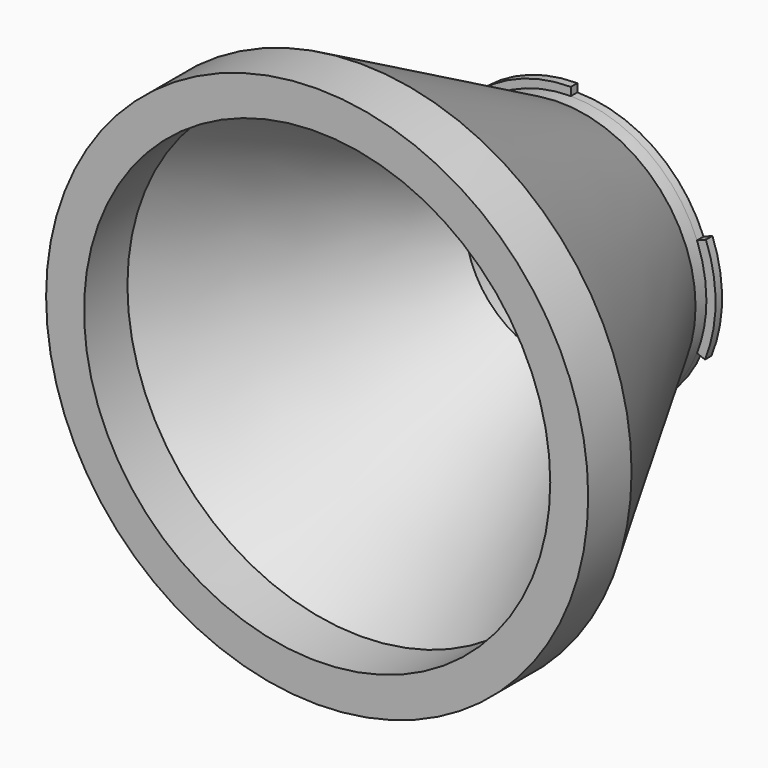
from build123d import *

# Parameters (mm, degrees)
F0_R      = 17.5
F1_DEPTH  = 1.5
F2_R      = 25
F2_R_2    = 17.5
F3_DEPTH  = 2.5
F6_R      = 50
F5_R      = 25
F9_R      = 17.5
F8_R      = 43
F11_R     = 50
F11_R_2   = 43
F12_DEPTH = 10


with BuildPart() as f1:
    # F0 (on Front) → F1 (new body)
    with BuildSketch(Plane.XZ):
        with BuildLine():
            ThreePointArc((23.2602203248, -9.1630862947), (24.5612042469, -4.663394251), (25, 0))
            ThreePointArc((25, 0), (24.5634220452, 4.651698338), (23.2689362058, 9.1409303603))
            ThreePointArc((23.2689362058, 9.1409303603), (14.0797148585, 20.6582097362), (0, 25))
            ThreePointArc((0, 25), (-10.9669811321, 22.4660927811), (-19.7108172513, 15.3780259879))
            ThreePointArc((-19.7108172513, 15.3780259879), (-24.9555737451, 1.4897446272), (-21.4003229393, -12.9238608046))
            ThreePointArc((-21.4003229393, -12.9238608046), (-12.2862418967, -21.7726493578), (0, -25))
            ThreePointArc((0, -25), (14.0698763789, -20.6649117754), (23.2602203248, -9.1630862947))
        make_face()
        Circle(F0_R, mode=Mode.SUBTRACT)
        with BuildLine():
            ThreePointArc((23.2689362058, 9.1409303603), (24.5634220452, 4.651698338), (25, 0))
            ThreePointArc((25, 0), (24.5612042469, -4.663394251), (23.2602203248, -9.1630862947))
            Line((23.2602203248, -9.1630862947), (24.7313799339, -9.7426320713))
            ThreePointArc((24.7313799339, -9.7426320713), (26.6870958696, 0.0047625742), (24.9132933265, 9.7868968881))
            Line((24.9132933265, 9.7868968881), (23.2689362058, 9.1409303603))
        make_face()
        with BuildLine():
            ThreePointArc((-19.7108172513, 15.3780259879), (-10.9669811321, 22.4660927811), (0, 25))
            Line((0, 25), (0, 26.5))
            ThreePointArc((0, 26.5), (-11.625, 23.814058348), (-20.8934662864, 16.3007075472))
            Line((-20.8934662864, 16.3007075472), (-19.7108172513, 15.3780259879))
        make_face()
        with BuildLine():
            Line((0, -26.7237641467), (0, -25))
            ThreePointArc((0, -25), (-12.2862418967, -21.7726493578), (-21.4003229393, -12.9238608046))
            Line((-21.4003229393, -12.9238608046), (-22.6843423156, -13.6992924528))
            ThreePointArc((-22.6843423156, -13.6992924528), (-13.0611614327, -23.205443504), (0, -26.7237641467))
        make_face()
    extrude(amount=F1_DEPTH)

    # F2 (on face) → F3 (join)
    with BuildSketch(Plane.XZ.offset(1.5)):
        Circle(F2_R)
        Circle(F2_R_2, mode=Mode.SUBTRACT)
    extrude(amount=F3_DEPTH)

    # F6 (on offset) → F7 section 0
    with BuildSketch(Plane.XZ.offset(50)):
        Circle(F6_R)
    # F5 (on face) → F7 section 1
    with BuildSketch(Plane.XZ.offset(4)):
        Circle(F5_R)
    loft()

    # F9 (on face) → F10 section 0
    with BuildSketch(Plane(origin=(0, -4, 0), x_dir=(-1, 0, 0), z_dir=(0, 1, 0))):
        Circle(F9_R)
    # F8 (on face) → F10 section 1
    with BuildSketch(Plane.XZ.offset(50)):
        Circle(F8_R)
    loft(mode=Mode.SUBTRACT)

    # F11 (on face) → F12 (join)
    with BuildSketch(Plane.XZ.offset(50)):
        Circle(F11_R)
        Circle(F11_R_2, mode=Mode.SUBTRACT)
    extrude(amount=F12_DEPTH)


solid = f1.part
